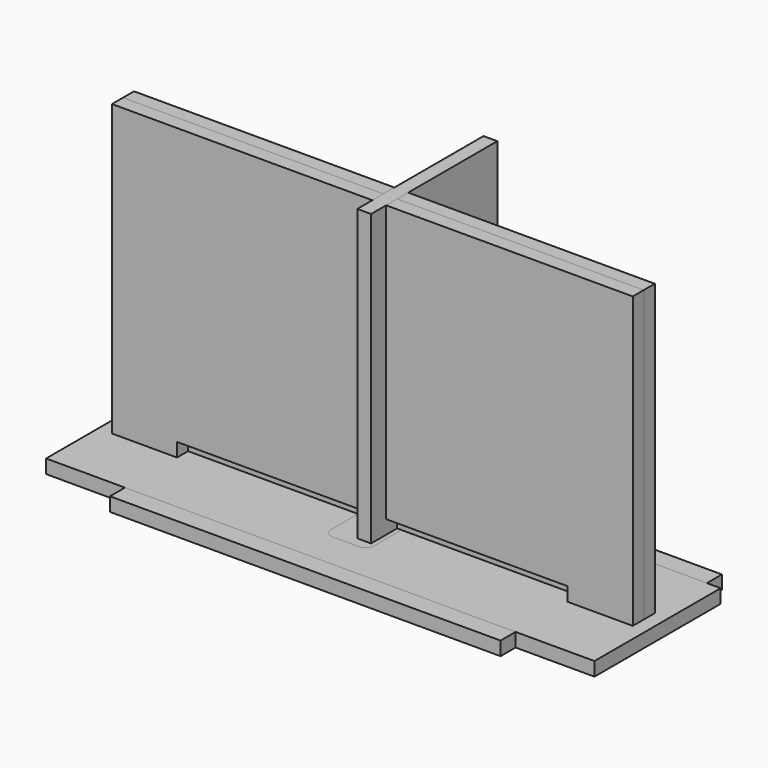
from build123d import *

# Parameters (mm, degrees)
F0_W     = 15
F0_H     = 30
F0_W_2   = 5
F0_H_2   = 5
F1_DEPTH = 3.175
F3_DEPTH = 3.175
F2_W     = 90
F2_H     = 6.35
F4_DEPTH = 3.175
F5_W     = 36.35
F5_H     = 70
F6_DEPTH = 3.175
F7_W     = 126.35
F7_H     = 36.35
F7_W_2   = 10
F7_H_2   = 20
F8_DEPTH = 3.175
F9_R     = 2


# Not quite as in the source:
# - a feature names something its author has since deleted; it is built from what else it names


with BuildPart() as f1:
    # F0 (on Top) → F1 (new body)
    with BuildSketch(Plane.XY):
        with Locations((52.5, 7.5)):
            Rectangle(F0_W, F0_H)
        with Locations((-52.5, 7.5)):
            Rectangle(F0_W, F0_H)
        Polygon((-45, -22.5), (45, -22.5), (45, -7.5), (45, 22.5), (-45, 22.5), (-45, -7.5), (-45, -10.675), align=None)
        with Locations((-35, 5)):
            Rectangle(F0_W_2, F0_H_2, mode=Mode.SUBTRACT)
        with Locations((-27.5, 5)):
            Rectangle(F0_W_2, F0_H_2, mode=Mode.SUBTRACT)
        with Locations((-20, 5)):
            Rectangle(F0_W_2, F0_H_2, mode=Mode.SUBTRACT)
        with Locations((-12.5, 5)):
            Rectangle(F0_W_2, F0_H_2, mode=Mode.SUBTRACT)
        with Locations((-5, 5)):
            Rectangle(F0_W_2, F0_H_2, mode=Mode.SUBTRACT)
        with Locations((2.5, 5)):
            Rectangle(F0_W_2, F0_H_2, mode=Mode.SUBTRACT)
        with Locations((10, 5)):
            Rectangle(F0_W_2, F0_H_2, mode=Mode.SUBTRACT)
        with Locations((17.5, 5)):
            Rectangle(F0_W_2, F0_H_2, mode=Mode.SUBTRACT)
        with Locations((25, 5)):
            Rectangle(F0_W_2, F0_H_2, mode=Mode.SUBTRACT)
        with Locations((32.5, 5)):
            Rectangle(F0_W_2, F0_H_2, mode=Mode.SUBTRACT)
    extrude(amount=F1_DEPTH)


with BuildPart() as f3:
    # F2 (on Front) → F3 (new body)
    with BuildSketch(Plane.XZ):
        Polygon((-60, 70), (-60, 0), (-45, 0), (-45, 6.35), (45, 6.35), (45, 0), (60, 0), (60, 70), align=None)
    extrude(amount=F3_DEPTH)


with BuildPart() as f4:
    # F2 (on Front) → F4 (new body)
    with BuildSketch(Plane.XZ):
        Polygon((-60, 70), (-60, 0), (-45, 0), (-45, 6.35), (45, 6.35), (45, 0), (60, 0), (60, 70), align=None)
        with Locations((0, 3.175)):
            Rectangle(F2_W, F2_H)
    extrude(amount=-F4_DEPTH)


with BuildPart() as f6:
    # F5 (on Right) → F6 (new body)
    with BuildSketch(Plane.YZ):
        with Locations((10.6640724358, 35)):
            Rectangle(F5_W, F5_H)
    extrude(amount=F6_DEPTH)


with BuildPart() as f8:
    # F7 (on Top) → F8 (new body)
    with BuildSketch(Plane.XY):
        Rectangle(F7_W, F7_H)
        with Locations((-0.825, 0.175)):
            Rectangle(F7_W_2, F7_H_2, mode=Mode.SUBTRACT)
    extrude(amount=F8_DEPTH)

    # F9
    f9_edges = [f8.edges().sort_by_distance(p)[0] for p in [
        (-5.825, 10.175, 1.5875),
        (4.175, 10.175, 1.5875),
        (4.175, -9.825, 1.5875),
        (-5.825, -9.825, 1.5875),
    ]]
    fillet(f9_edges, radius=F9_R)


solid = Compound([f1.part, f3.part, f4.part, f6.part, f8.part])
